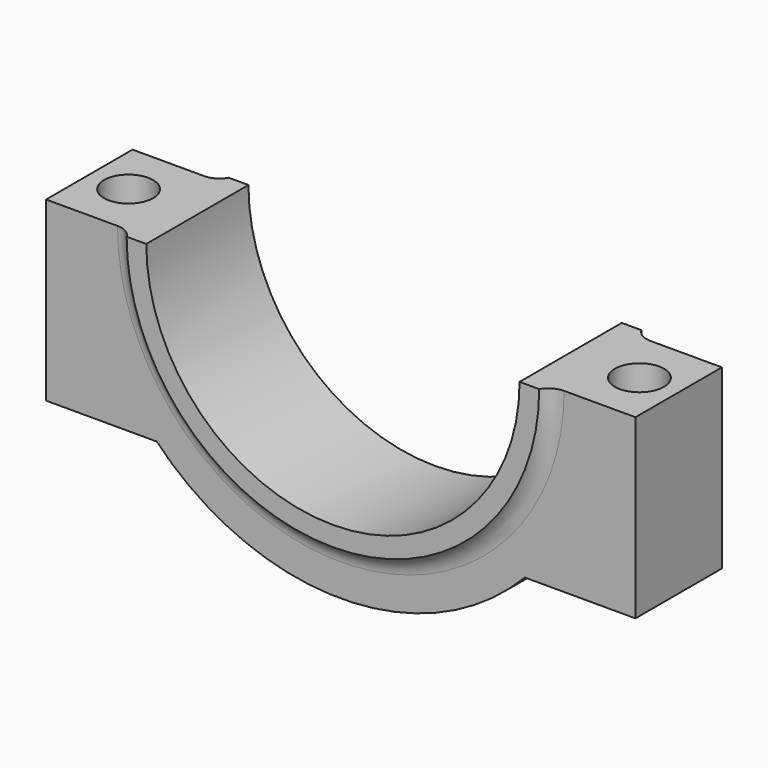
from build123d import *

# Parameters (mm, degrees)
F1_DEPTH    = 5.5
F2_DEPTH    = 6.5
F3_T2_ANGLE = 180
F3_T4_ANGLE = 180
F4_R        = 2.5
F5_DEPTH    = 25.4


# Not quite as in the source:
# - a fillet or chamfer that OpenCascade refuses, or shapes differently, is made with other operations: its cross-section is extruded or revolved along the edge and cut away or added


with BuildPart() as f1:
    # F0 (on Front) → F1 (new body, symmetric)
    with BuildSketch(Plane.XZ):
        with BuildLine():
            ThreePointArc((19, 0), (0, -19), (-19, 0))
            Line((-19, 0), (-21, 0))
            ThreePointArc((-21, 0), (0, -21), (21, 0))
            Line((21, 0), (19, 0))
        make_face()
        with BuildLine():
            ThreePointArc((21, 0), (0, -21), (-21, 0))
            Line((-21, 0), (-30, 0))
            Line((-30, 0), (-30, -18.0277563773))
            Line((-30, -18.0277563773), (-18.7349939952, -18.0277563773))
            ThreePointArc((-18.7349939952, -18.0277563773), (0, -26), (18.7349939952, -18.0277563773))
            Line((18.7349939952, -18.0277563773), (30, -18.0277563773))
            Line((30, -18.0277563773), (30, 0))
            Line((30, 0), (21, 0))
        make_face()
    extrude(amount=F1_DEPTH, both=True)

    # F0 (on Front) → F2 (join, symmetric)
    with BuildSketch(Plane.XZ):
        with BuildLine():
            ThreePointArc((19, 0), (0, -19), (-19, 0))
            Line((-19, 0), (-21, 0))
            ThreePointArc((-21, 0), (0, -21), (21, 0))
            Line((21, 0), (19, 0))
        make_face()
    extrude(amount=F2_DEPTH, both=True)

    # F3: fillet of radius 2 on 2 edges, made by hand

    # F3_s1 → F3_t2 (revolve)
    with BuildSketch(Plane.XY):
        with BuildLine():
            ThreePointArc((-22.7320508076, 5.5), (-21.7320508076, 5.7679491924), (-21, 6.5))
            Line((-21, 6.5), (-21, 5.5))
            Line((-21, 5.5), (-22.7320508076, 5.5))
        make_face()
    revolve(axis=Axis((0, 5.5, 0), (0, -1, 0)), revolution_arc=F3_T2_ANGLE)

    # F3_s3 → F3_t4 (revolve)
    with BuildSketch(Plane.XY):
        with BuildLine():
            ThreePointArc((-21, -6.5), (-21.7320508076, -5.7679491924), (-22.7320508076, -5.5))
            Line((-22.7320508076, -5.5), (-21, -5.5))
            Line((-21, -5.5), (-21, -6.5))
        make_face()
    revolve(axis=Axis((0, -5.5, 0), (0, -1, 0)), revolution_arc=F3_T4_ANGLE)

    # F4 (on Top) → F5 (cut)
    with BuildSketch(Plane.XY):
        with Locations((-26, 0)):
            Circle(F4_R)
        with Locations((26, 0)):
            Circle(F4_R)
    extrude(amount=-F5_DEPTH, mode=Mode.SUBTRACT)


solid = f1.part
